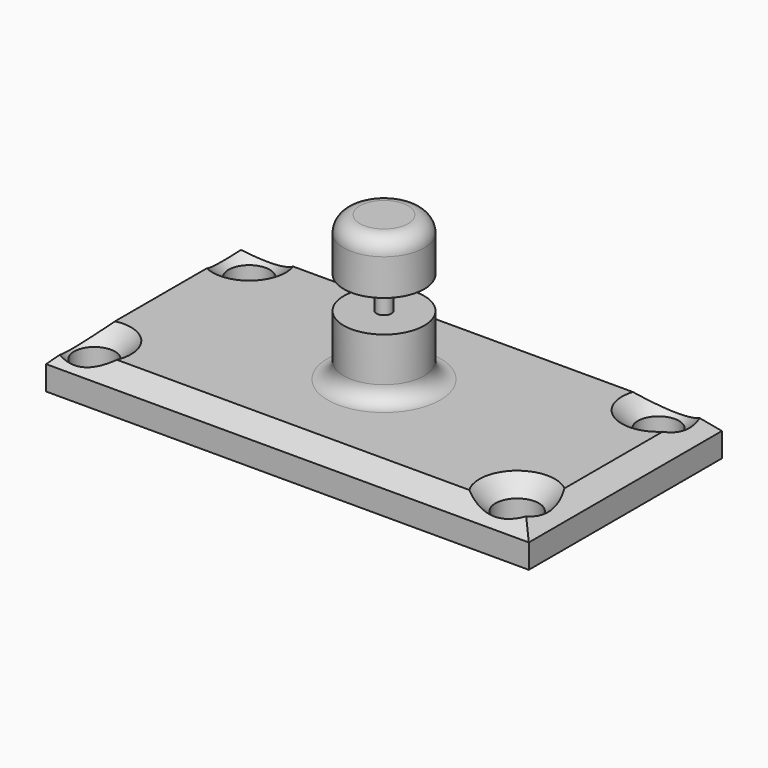
from build123d import *

# Parameters (mm, degrees)
F1_DEPTH     = 12.7
F3_R         = 7.826189497
F3_R_2       = 7.6449247614
F3_R_3       = 9.3914167861
F3_R_4       = 7.5169302634
F2_R         = 6.8354514468
F2_R_2       = 6.4833469735
F2_R_3       = 6.4699307045
F2_R_4       = 6.483339071
F4_DEPTH     = 25.4
F5_W         = 12.7
F5_H         = 45.72
F7_W         = 12.7
F7_H         = 10.16
F9_R         = 5.08
F10_T1_DEPTH = 102.3282991577
F10_T3_DEPTH = 178.5282991577


# Not quite as in the source:
# - a fillet or chamfer that OpenCascade refuses, or shapes differently, is made with other operations: its cross-section is extruded or revolved along the edge and cut away or added


with BuildPart() as f1:
    # F0 (on Top) → F1 (new body)
    with BuildSketch(Plane.XY):
        Polygon((76.2, 21.421205096), (76.2, 38.1), (-76.2, 38.1), (-76.2, -38.1), (76.2, -38.1), align=None)
    extrude(amount=F1_DEPTH)

    # F3 (on face) + F2 (on face) → F4 (cut)
    with BuildSketch(Plane.XY):
        with Locations((-66.4894506335, 28.616681695)):
            Circle(F3_R)
        with Locations((60.850225389, 29.538076371)):
            Circle(F3_R_2)
        with Locations((62.7190470695, -24.263875559)):
            Circle(F3_R_3)
        with Locations((-67.1401694417, -24.8782932758)):
            Circle(F3_R_4)
    with BuildSketch(Plane.XY.offset(12.7)):
        with Locations((63.5566338897, -26.8813353032)):
            Circle(F2_R)
        with Locations((63.1398707628, 29.3819215149)):
            Circle(F2_R_2)
        with Locations((-68.5578212142, -28.5483933985)):
            Circle(F2_R_3)
        with Locations((-66.0572275519, 29.3819215149)):
            Circle(F2_R_4)
    extrude(amount=-F4_DEPTH, mode=Mode.SUBTRACT)

    # F5 (on Front) → F6 (revolve)
    with BuildSketch(Plane.XZ):
        with Locations((6.35, 35.56)):
            Rectangle(F5_W, F5_H)
    revolve(axis=Axis((0, 0, 35.56), (0, 0, -1)))

    # F7 (on Front) → F8 (revolve, cut)
    with BuildSketch(Plane.XZ):
        with Locations((8.7274818003, 36.8085707384)):
            Rectangle(F7_W, F7_H)
    revolve(axis=Axis((0, 0, 12.7), (0, 0, 1)), mode=Mode.SUBTRACT)

    # F9
    f9_edges = [f1.edges().sort_by_distance(p)[0] for p in [
        (-12.7, 0, 58.42),
        (-12.7, 0, 12.7),
    ]]
    fillet(f9_edges, radius=F9_R)

    # F10: chamfer of 5.08 on 9 edges, made by hand

    # F10_s2 → F10_t1 (cut)
    with BuildSketch(Plane.XZ.offset(-51.1641495789)):
        Polygon((71.12, 12.7), (76.2, 7.62), (76.2, 12.7), align=None)
        Polygon((-71.12, 12.7), (-76.2, 7.62), (-76.2, 12.7), align=None)
    extrude(amount=F10_T1_DEPTH, mode=Mode.SUBTRACT)

    # F10_s4 → F10_t3 (cut)
    with BuildSketch(Plane.YZ.offset(-89.2641495789)):
        Polygon((33.02, 12.7), (38.1, 7.62), (38.1, 12.7), align=None)
        Polygon((-33.02, 12.7), (-38.1, 7.62), (-38.1, 12.7), align=None)
    extrude(amount=F10_T3_DEPTH, mode=Mode.SUBTRACT)

    # F10_s5 → F10_t6 (revolve, cut)
    with BuildSketch(Plane.XZ.offset(28.5483933985)):
        Polygon((-57.0078905097, 12.7), (-62.0878905097, 7.62), (-62.0878905097, 12.7), align=None)
    revolve(axis=Axis((-68.5578212142, -28.5483933985, 12.7), (0, 0, 1)), mode=Mode.SUBTRACT)

    # F10_s7 → F10_t8 (revolve, cut)
    with BuildSketch(Plane.XZ.offset(26.8813353032)):
        Polygon((75.4720853364, 12.7), (70.3920853364, 7.62), (70.3920853364, 12.7), align=None)
    revolve(axis=Axis((63.5566338897, -26.8813353032, 12.7), (0, 0, 1)), mode=Mode.SUBTRACT)

    # F10_s9 → F10_t10 (revolve, cut)
    with BuildSketch(Plane.XZ.offset(-29.3819215149)):
        Polygon((-54.493888481, 12.7), (-59.573888481, 7.62), (-59.573888481, 12.7), align=None)
    revolve(axis=Axis((-66.0572275519, 29.3819215149, 12.7), (0, 0, 1)), mode=Mode.SUBTRACT)

    # F10_s11 → F10_t12 (revolve, cut)
    with BuildSketch(Plane.XZ.offset(-29.3819215149)):
        Polygon((74.7032177363, 12.7), (69.6232177363, 7.62), (69.6232177363, 12.7), align=None)
    revolve(axis=Axis((63.1398707628, 29.3819215149, 12.7), (0, 0, 1)), mode=Mode.SUBTRACT)


solid = f1.part
